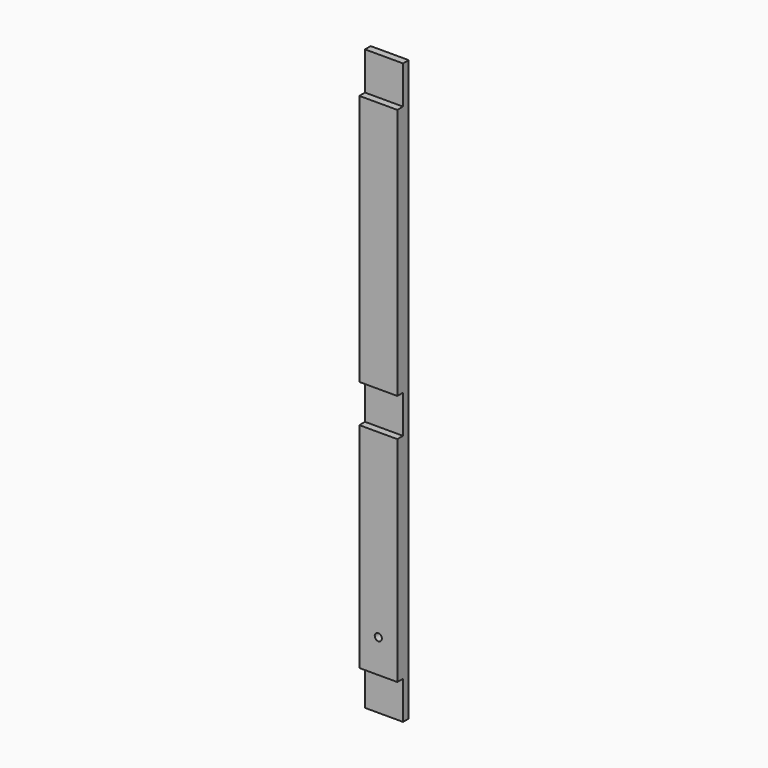
from build123d import *

# Parameters (mm, degrees)
F0_W     = 50.8
F0_H     = 19.05
F1_DEPTH = 774.7
F2_W     = 122.43557321
F2_H     = 50.8
F2_W_2   = 343.1604206562
F2_W_3   = 296.3738366961
F3_DEPTH = 25.4
F4_R     = 0.79375
F5_DEPTH = 25.4
F6_R     = 4.7625
F7_DEPTH = 25.4


# Not quite as in the source:
# - a feature names something its author has since deleted; it is built from what else it names


with BuildPart() as f1:
    # F0 (on Top) → F1 (new body)
    with BuildSketch(Plane.XY):
        Rectangle(F0_W, F0_H)
    extrude(amount=F1_DEPTH)

    # F2 (on Front) → F3 (cut)
    with BuildSketch(Plane.XZ):
        with Locations((22.4465244144, 25.4)):
            Rectangle(F2_W, F2_H)
        with Locations((-38.7818217278, 749.3)):
            Rectangle(F2_W_2, F2_H)
        with Locations((-46.0684634745, 361.95)):
            Rectangle(F2_W_3, F2_H)
    extrude(amount=F3_DEPTH, mode=Mode.SUBTRACT)

    # F4 (on Front) → F5 (cut)
    with BuildSketch(Plane.XZ):
        with Locations((9.525, 101.6)):
            Circle(F4_R)
        with Locations((9.525, 155.575)):
            Circle(F4_R)
        with Locations((9.525, 517.525)):
            Circle(F4_R)
        with Locations((9.525, 571.5)):
            Circle(F4_R)
        with Locations((-9.525, 517.525)):
            Circle(F4_R)
        with Locations((-9.525, 571.5)):
            Circle(F4_R)
        with Locations((-9.525, 101.6)):
            Circle(F4_R)
        with Locations((-9.525, 155.575)):
            Circle(F4_R)
    extrude(amount=-F5_DEPTH, mode=Mode.SUBTRACT)

    # F6 (on Front) → F7 (cut)
    with BuildSketch(Plane.XZ):
        with Locations((0, 95.25)):
            Circle(F6_R)
        with Locations((0, 361.95)):
            Circle(F6_R)
    extrude(amount=F7_DEPTH, mode=Mode.SUBTRACT)


solid = f1.part
